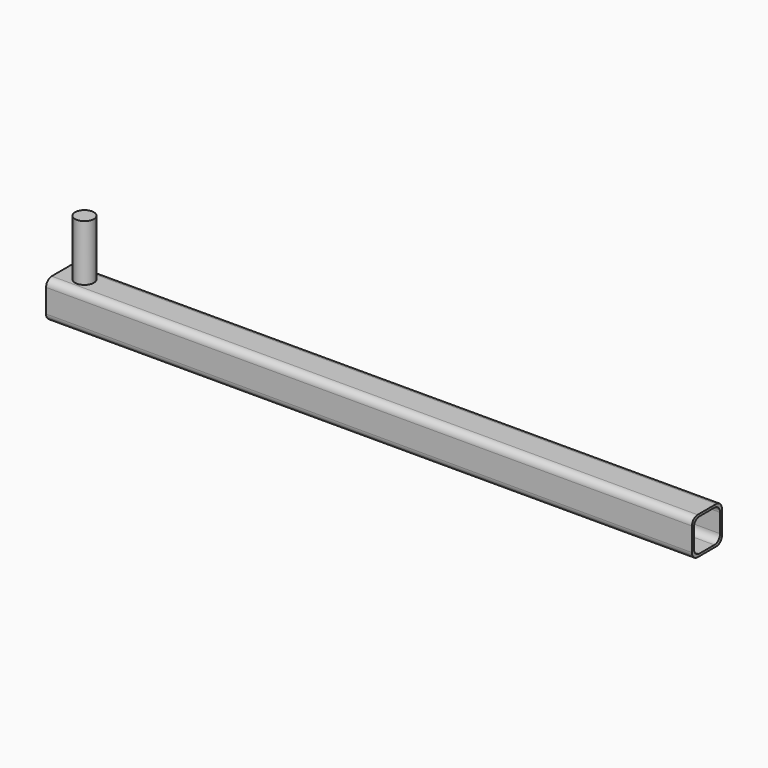
from build123d import *

# Parameters (mm, degrees)
F0_W     = 50.8
F0_H     = 50.8
F1_DEPTH = 876.3
F2_W     = 44.45
F2_H     = 44.45
F3_DEPTH = 876.3
F4_R     = 9.525
F5_R     = 12.7
F6_DEPTH = 50.8
F7_R     = 12.7
F8_DEPTH = 127


with BuildPart() as f1:
    # F0 (on Right) → F1 (new body)
    with BuildSketch(Plane.YZ):
        with Locations((25.4, 25.4)):
            Rectangle(F0_W, F0_H)
    extrude(amount=-F1_DEPTH)

    # F2 (on face) → F3 (cut)
    with BuildSketch(Plane.YZ):
        with Locations((25.4, 25.4)):
            Rectangle(F2_W, F2_H)
    extrude(amount=-F3_DEPTH, mode=Mode.SUBTRACT)

    # F4
    f4_edges = [f1.edges().sort_by_distance(p)[0] for p in [
        (-438.15, 3.175, 3.175),
        (-438.15, 47.625, 3.175),
        (-438.15, 47.625, 47.625),
        (-438.15, 3.175, 47.625),
        (-438.15, 50.8, 0),
        (-438.15, 50.8, 50.8),
        (-438.15, 0, 50.8),
        (-438.15, 0, 0),
    ]]
    fillet(f4_edges, radius=F4_R)

    # F5 (on face) → F6 (cut)
    with BuildSketch(Plane.XY.offset(50.8)):
        with Locations((-844.55, 25.4)):
            Circle(F5_R)
    extrude(amount=-F6_DEPTH, mode=Mode.SUBTRACT)

    # F7 (on face) → F8 (join)
    with BuildSketch(Plane(origin=(0, 0, 0), x_dir=(1, 0, 0), z_dir=(0, 0, -1))):
        with Locations((-844.55, -25.4)):
            Circle(F7_R)
    extrude(amount=-F8_DEPTH)


solid = f1.part
